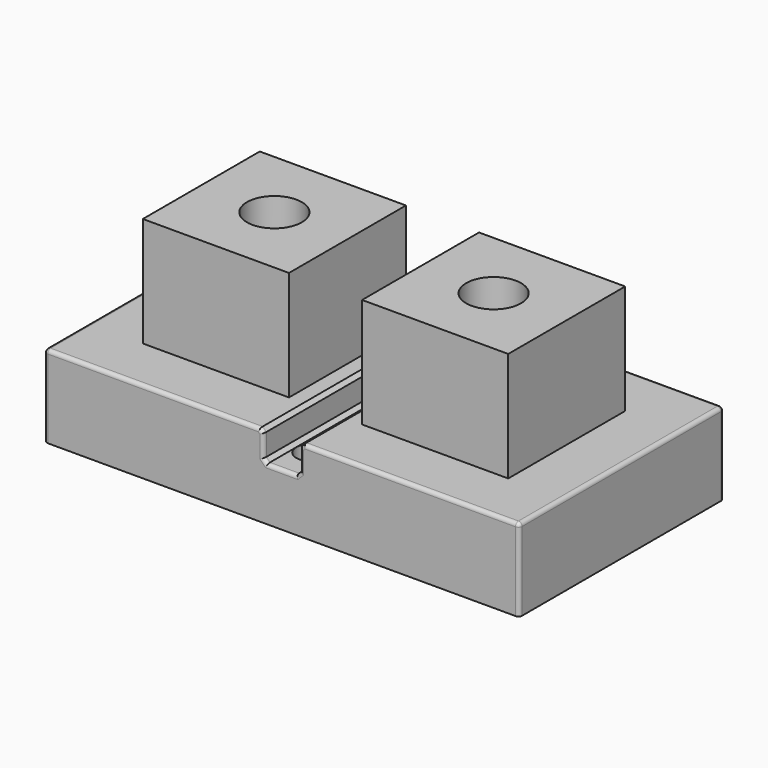
from build123d import *

# Parameters (mm, degrees)
F0_W     = 25.4
F0_H     = 25.4
F0_R     = 4.7625
F0_W_2   = 3.175
F0_W_3   = 6.35
F0_R_2   = 2.54
F1_DEPTH = 14.2875
F2_DEPTH = 19.05
F3_DEPTH = 5.08
F4_DEPTH = 14.2875
F5_SIZE  = 0.63499
F6_R     = 0.635


# Not quite as in the source:
# - a fillet or chamfer is up to 0.001 mm smaller than in the source, because OpenCascade refuses the exact size
# - a feature names something its author has since deleted; it is built from what else it names


with BuildPart() as f1:
    # F0 (on Top) → F1 (new body)
    with BuildSketch(Plane.XY):
        Polygon((-6.35, 12.7), (-3.175, 12.7), (-3.175, 22.225), (-41.275, 22.225), (-41.275, -22.225), (-3.175, -22.225), (-3.175, -12.7), (-6.35, -12.7), (-31.75, -12.7), (-31.75, 12.7), align=None)
        with Locations((-19.05, 0)):
            Rectangle(F0_W, F0_H)
        with Locations((-19.05, 0)):
            Circle(F0_R, mode=Mode.SUBTRACT)
        with Locations((-4.7625, 0)):
            Rectangle(F0_W_2, F0_H)
        Rectangle(F0_W_3, F0_H)
        Polygon((3.175, 12.7), (3.175, 22.225), (2.54, 22.225), (-2.54, 22.225), (-3.175, 22.225), (-3.175, 12.7), align=None)
        with Locations((0, 15.875)):
            Circle(F0_R_2, mode=Mode.SUBTRACT)
        Polygon((2.54, -22.225), (3.175, -22.225), (3.175, -12.7), (-3.175, -12.7), (-3.175, -22.225), (-2.54, -22.225), align=None)
        with Locations((0, -15.875)):
            Circle(F0_R_2, mode=Mode.SUBTRACT)
        Polygon((41.275, -22.225), (41.275, 22.225), (3.175, 22.225), (3.175, 12.7), (6.35, 12.7), (31.75, 12.7), (31.75, -12.7), (6.35, -12.7), (3.175, -12.7), (3.175, -22.225), align=None)
        with Locations((4.7625, 0)):
            Rectangle(F0_W_2, F0_H)
        with Locations((19.05, 0)):
            Rectangle(F0_W, F0_H)
        with Locations((19.05, 0)):
            Circle(F0_R, mode=Mode.SUBTRACT)
        with Locations((19.05, 0)):
            Circle(F0_R)
        with Locations((-19.05, 0)):
            Circle(F0_R)
    extrude(amount=-F1_DEPTH)

    # F0 (on Top) → F2 (join)
    with BuildSketch(Plane.XY):
        with Locations((-19.05, 0)):
            Rectangle(F0_W, F0_H)
        with Locations((-19.05, 0)):
            Circle(F0_R, mode=Mode.SUBTRACT)
        with Locations((19.05, 0)):
            Rectangle(F0_W, F0_H)
        with Locations((19.05, 0)):
            Circle(F0_R, mode=Mode.SUBTRACT)
    extrude(amount=F2_DEPTH)

    # F0 (on Top) → F3 (cut)
    with BuildSketch(Plane.XY):
        Rectangle(F0_W_3, F0_H)
        Polygon((2.54, -22.225), (3.175, -22.225), (3.175, -12.7), (-3.175, -12.7), (-3.175, -22.225), (-2.54, -22.225), align=None)
        with Locations((0, -15.875)):
            Circle(F0_R_2, mode=Mode.SUBTRACT)
        Polygon((3.175, 12.7), (3.175, 22.225), (2.54, 22.225), (-2.54, 22.225), (-3.175, 22.225), (-3.175, 12.7), align=None)
        with Locations((0, 15.875)):
            Circle(F0_R_2, mode=Mode.SUBTRACT)
    extrude(amount=-F3_DEPTH, mode=Mode.SUBTRACT)

    # F0 (on Top) → F4 (cut)
    with BuildSketch(Plane.XY):
        with Locations((0, -15.875)):
            Circle(F0_R_2)
        with Locations((0, 15.875)):
            Circle(F0_R_2)
    extrude(amount=-F4_DEPTH, mode=Mode.SUBTRACT)

    # F5 (size 0.635 in the source; OpenCascade refuses exactly that, so slightly less here)
    f5_edges = [f1.edges().sort_by_distance(p)[0] for p in [
        (3.175, 0, -5.08),
        (-3.175, 0, -5.08),
        (3.175, 0, 0),
        (-3.175, 0, 0),
    ]]
    chamfer(f5_edges, length=F5_SIZE)

    # F6
    f6_edges = [f1.edges().sort_by_distance(p)[0] for p in [
        (-22.542495, -22.225, 0),
        (-3.492495, -22.225, -0.317495),
        (-2.857505, -22.225, -4.762505),
        (0, -22.225, -5.08),
        (2.857505, -22.225, -4.762505),
        (3.175, -22.225, -2.54),
        (3.492495, -22.225, -0.317495),
        (22.542495, -22.225, 0),
        (-41.275, -22.225, -7.14375),
        (-41.275, 0, 0),
        (-41.275, 22.225, -7.14375),
        (-22.542495, 22.225, 0),
        (-3.175, 22.225, -2.54),
        (-3.492495, 22.225, -0.317495),
        (0, 22.225, -5.08),
        (-2.857505, 22.225, -4.762505),
        (22.542495, 22.225, 0),
        (3.175, 22.225, -2.54),
        (3.492495, 22.225, -0.317495),
        (41.275, 22.225, -7.14375),
        (41.275, 0, 0),
        (41.275, -22.225, -7.14375),
        (2.857505, 22.225, -4.762505),
        (-3.175, -22.225, -2.54),
    ]]
    fillet(f6_edges, radius=F6_R)


solid = f1.part
